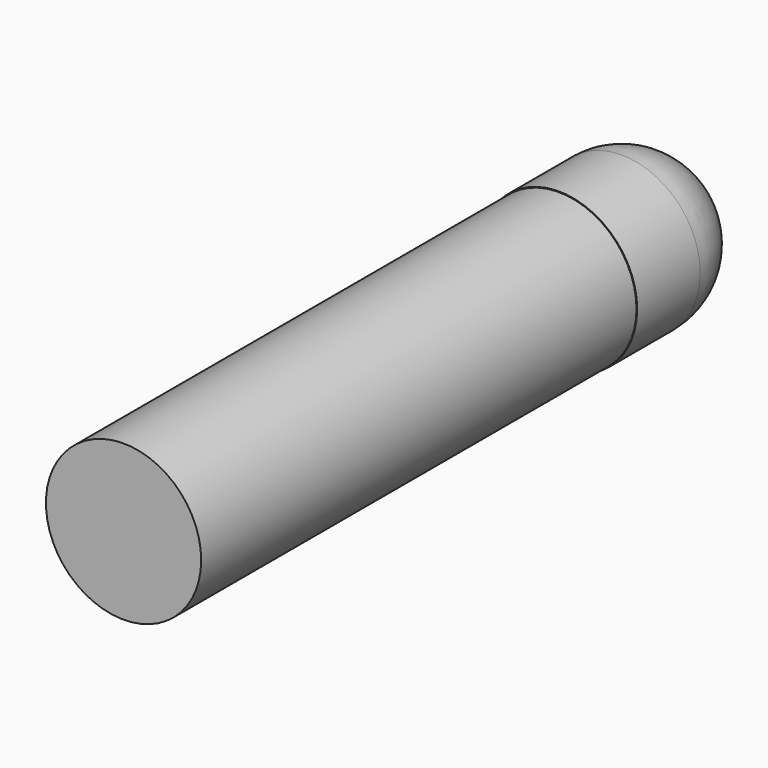
from build123d import *

# Parameters (mm, degrees)
F0_R     = 25.5877592178
F0_R_2   = 4.2037211277
F1_DEPTH = 50.8
F3_T     = -2.54
F4_R     = 25.3646729185
F5_DEPTH = 177.8


# Not quite as in the source:
# - a fillet or chamfer that OpenCascade refuses, or shapes differently, is made with other operations: its cross-section is extruded or revolved along the edge and cut away or added


with BuildPart() as f1:
    # F0 (on Front) → F1 (new body)
    with BuildSketch(Plane.XZ):
        Circle(F0_R)
        Circle(F0_R_2, mode=Mode.SUBTRACT)
    extrude(amount=F1_DEPTH)

    # F2: fillet of radius 25.4 on 1 edges, made by hand

    # F2_s1 → F2_t2 (revolve, cut)
    with BuildSketch(Plane.XY):
        with BuildLine():
            ThreePointArc((25.5877592178, -25.0805113572), (19.5160471982, -8.6009093067), (4.2037211277, 0))
            Line((4.2037211277, 0), (25.5877592178, 0))
            Line((25.5877592178, 0), (25.5877592178, -25.0805113572))
        make_face()
    revolve(axis=Axis((0, 0, 0), (0, -1, 0)), mode=Mode.SUBTRACT)

    # F3
    f3_openings = [f1.faces().sort_by_distance(p)[0] for p in [
        (-24.864028, -50.8, 0),
    ]]
    offset(amount=F3_T, openings=f3_openings, kind=Kind.INTERSECTION)

    # F4 (on face) → F5 (join)
    with BuildSketch(Plane.XZ.offset(50.8)):
        Circle(F4_R)
    extrude(amount=F5_DEPTH)


solid = f1.part
